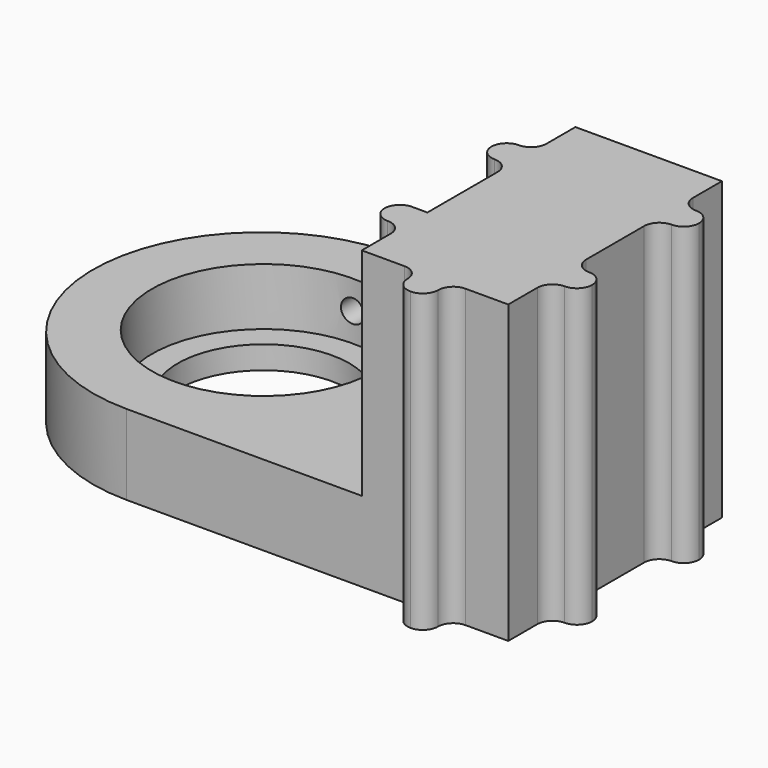
from build123d import *

# Parameters (mm, degrees)
F0_R      = 22
F0_R_2    = 11.25
F1_DEPTH  = 10.5
F3_DEPTH  = 38.82
F4_R      = 14.625
F4_R_2    = 11.125
F5_DEPTH  = 7.5
F8_W      = 13.208
F8_H      = 20.32
F9_DEPTH  = 32.5
F10_R     = 3
F11_DEPTH = 15.4999664724
F12_W     = 13.208
F12_H     = 30.5
F13_DEPTH = 1.5
F14_W     = 13.208
F14_H     = 30.5
F15_DEPTH = 1
F16_W     = 30.8
F16_H     = 28.32
F17_DEPTH = 44.001
F18_W     = 4
F18_H     = 4
F19_DEPTH = 38.82
F20_R     = 1.99999
F7_R      = 1.5
F21_DEPTH = 10


# Not quite as in the source:
# - a fillet or chamfer is up to 0.001 mm smaller than in the source, because OpenCascade refuses the exact size
# - a feature names something its author has since deleted; it is built from what else it names


with BuildPart() as f1:
    # F0 (on Top) → F1 (new body)
    with BuildSketch(Plane.XY):
        Circle(F0_R)
        with Locations((-1.609e-06, 0.4174434871)):
            Circle(F0_R_2, mode=Mode.SUBTRACT)
    extrude(amount=F1_DEPTH)

    # F2 (on Top) → F3 (join)
    with BuildSketch(Plane.XY):
        with BuildLine():
            Line((0, -22), (50, -22))
            Line((50, -22), (50, 13))
            Line((50, 13), (17.7482393493, 13))
            ThreePointArc((17.7482393493, 13), (19.6214168703, -9.9498743711), (0, -22))
        make_face()
    extrude(amount=F3_DEPTH)

    # F4 (on face) → F5 (cut)
    with BuildSketch(Plane.XY.offset(10.5)):
        with Locations((-1.609e-06, 0.4174434871)):
            Circle(F4_R)
        with Locations((-1.609e-06, 0.4174434871)):
            Circle(F4_R_2, mode=Mode.SUBTRACT)
    extrude(amount=-F5_DEPTH, mode=Mode.SUBTRACT)

    # F8 (on face) → F9 (cut)
    with BuildSketch(Plane(origin=(0, 13, 0), x_dir=(-1, 0, 0), z_dir=(0, 1, 0))):
        with Locations((-40.396, 25.6599664724)):
            Rectangle(F8_W, F8_H)
    extrude(amount=-F9_DEPTH, mode=Mode.SUBTRACT)

    # F10 (on face) → F11 (cut, through all)
    with BuildSketch(Plane.XY.offset(15.4999664724)):
        with Locations((40.396, -15.5)):
            Circle(F10_R)
    extrude(amount=-F11_DEPTH, mode=Mode.SUBTRACT)

    # F12 (on face) → F13 (cut)
    with BuildSketch(Plane.XY.offset(15.4999664724)):
        with Locations((40.396, -4.25)):
            Rectangle(F12_W, F12_H)
    extrude(amount=-F13_DEPTH, mode=Mode.SUBTRACT)

    # F14 (on face) → F15 (cut)
    with BuildSketch(Plane(origin=(0, 0, 35.8199664724), x_dir=(1, 0, 0), z_dir=(0, 0, -1))):
        with Locations((40.396, 4.25)):
            Rectangle(F14_W, F14_H)
    extrude(amount=-F15_DEPTH, mode=Mode.SUBTRACT)

    # F16 (on face) → F17 (cut, through all)
    with BuildSketch(Plane.XZ.offset(22)):
        with Locations((15.4, 24.66)):
            Rectangle(F16_W, F16_H)
    extrude(amount=-F17_DEPTH, mode=Mode.SUBTRACT)

    # F18 (on face) → F19 (join, through all)
    with BuildSketch(Plane.XY.offset(38.82)):
        with Locations((52, 4.25)):
            Rectangle(F18_W, F18_H)
        with Locations((52, -13.25)):
            Rectangle(F18_W, F18_H)
        with Locations((28.8, -13.25)):
            Rectangle(F18_W, F18_H)
        with Locations((28.8, 4.25)):
            Rectangle(F18_W, F18_H)
        Polygon((40.4, -22), (38.4, -22), (38.4, -26), (42.4, -26), (42.4, -22), align=None)
    extrude(amount=-F19_DEPTH)

    # F20 (radius 2 in the source; OpenCascade refuses exactly that, so slightly less here)
    f20_edges = [f1.edges().sort_by_distance(p)[0] for p in [
        (42.4, -26, 19.41),
        (38.4, -26, 19.41),
        (42.4, -22, 19.41),
        (50, -15.25, 19.41),
        (54, -15.25, 19.41),
        (54, -11.25, 19.41),
        (50, 2.25, 19.41),
        (54, 2.25, 19.41),
        (54, 6.25, 19.41),
        (26.8, 2.25, 24.66),
        (26.8, -15.25, 24.66),
        (50, -11.25, 19.41),
        (50, 6.25, 19.41),
        (38.4, -22, 19.41),
        (26.8, -11.25, 24.66),
        (26.8, 6.25, 24.66),
        (30.8, 6.25, 24.66),
        (30.8, 2.25, 24.66),
        (30.8, -15.25, 24.66),
    ]]
    fillet(f20_edges, radius=F20_R)

    # F7 (on offset) → F21 (cut)
    with BuildSketch(Plane.XZ.offset(-22)):
        with Locations((0, 6.75)):
            Circle(F7_R)
    extrude(amount=F21_DEPTH, mode=Mode.SUBTRACT)


solid = f1.part
